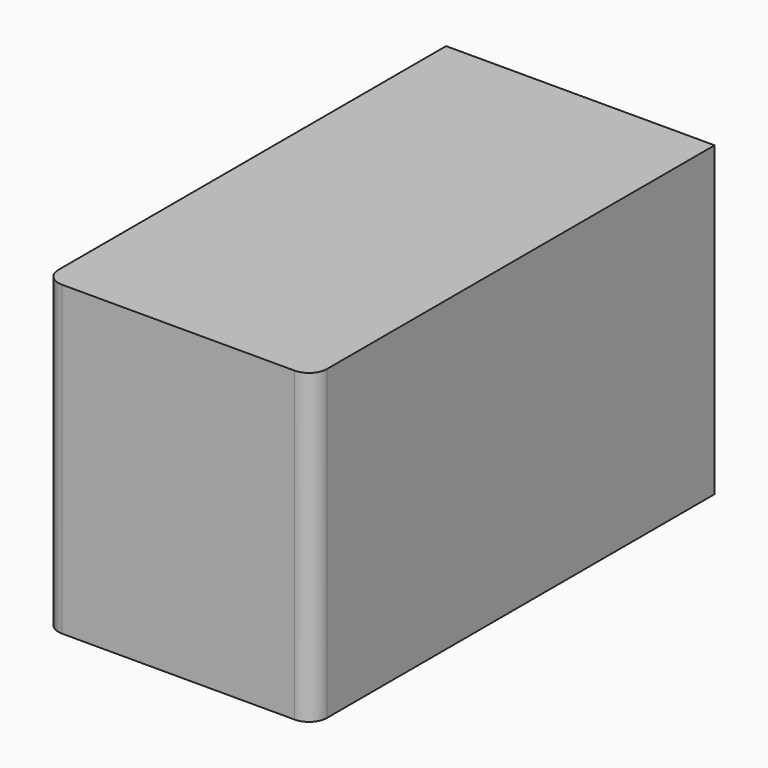
from build123d import *

# Parameters (mm, degrees)
F2_W     = 142.5837241113
F2_H     = 87.1813744307
F3_DEPTH = 76.2
F4_R     = 5.08


# Not quite as in the source:
# - a feature of the source that left no trace in its solid (it failed there, or was rolled back) is left out


with BuildPart() as f3:
    # F2 (on Right) → F3 (new body)
    with BuildSketch(Plane.YZ):
        with Locations((-24.0451861173, -18.1393511593)):
            Rectangle(F2_W, F2_H)
    extrude(amount=F3_DEPTH)

    # F4
    f4_edges = [f3.edges().sort_by_distance(p)[0] for p in [
        (0, -95.337048, -18.139351),
        (76.2, -95.337048, -18.139351),
    ]]
    fillet(f4_edges, radius=F4_R)


solid = f3.part
